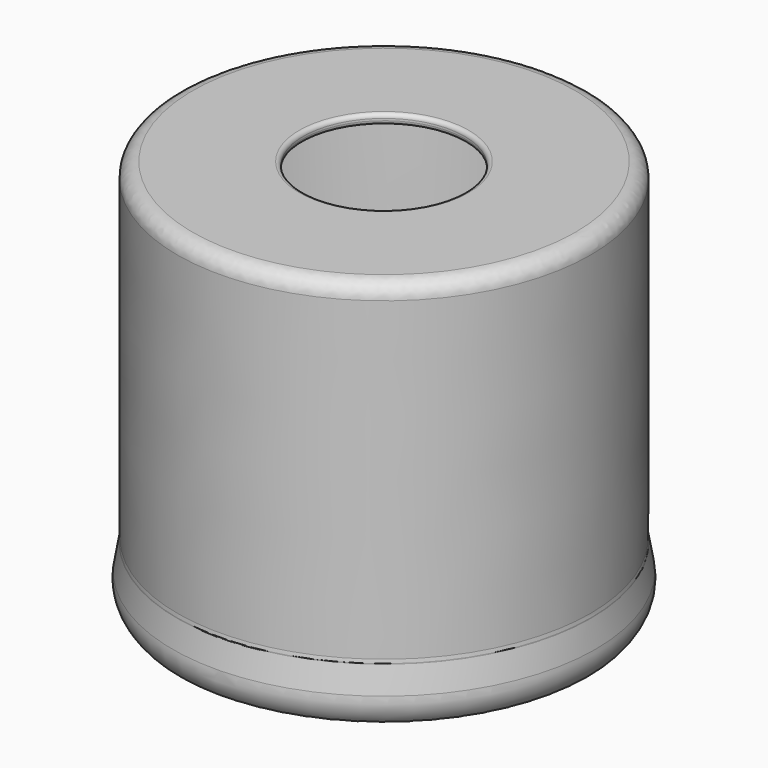
from build123d import *

# Parameters (mm, degrees)
F2_R = 1.5


# Not quite as in the source:
# - a feature names something its author has since deleted; it is built from what else it names


with BuildPart() as f1:
    # F0 (on Front) → F1 (revolve)
    with BuildSketch(Plane.XZ):
        with BuildLine():
            Line((19.479055467, 4.704423259), (20, 1.75))
            ThreePointArc((20, 1.75), (19.9515705454, 0.8174084156), (19.5, 0))
            ThreePointArc((19.5, 0), (19.5383526697, -0.7060657035), (20.2444183958, -0.6677134505))
            ThreePointArc((20.2444183958, -0.6677134505), (20.9130939683, 0.5426865853), (20.9848072317, 1.9236472929))
            Line((20.9848072317, 1.9236472929), (20.5337021691, 4.4819912332))
            Line((20.5337021691, 4.4819912332), (20.4790552528, 4.7037687424))
            Line((20.4790552528, 4.7037687424), (20.5000002142, 36.7044164045))
            Line((20.5000002142, 36.7044164048), (20.5000002142, 37.7044164048))
            Line((20.5000002142, 37.7044164048), (8.4, 37.7044164048))
            ThreePointArc((8.4, 37.7044164048), (8.1171572875, 37.5872591172), (8, 37.3044164048))
            Line((8, 37.3044164048), (8, 37.1044164048))
            ThreePointArc((8, 37.1044164048), (8.1171572875, 36.8215736923), (8.4, 36.7044164048))
            Line((8.4, 36.7044164048), (19.5, 36.7044164048))
            Line((19.5, 36.7044164048), (19.479055467, 4.704423259))
        make_face()
    revolve(axis=Axis((0, 0, 24.7507560998), (0, 0, 1)))

    # F2
    f2_edges = [f1.edges().sort_by_distance(p)[0] for p in [
        (-20.5, 0, 37.704416),
        (-19.5, 0, 36.704416),
        (-20.479055, 0, 4.703769),
        (-19.479055, 0, 4.704423),
    ]]
    fillet(f2_edges, radius=F2_R)


solid = f1.part
